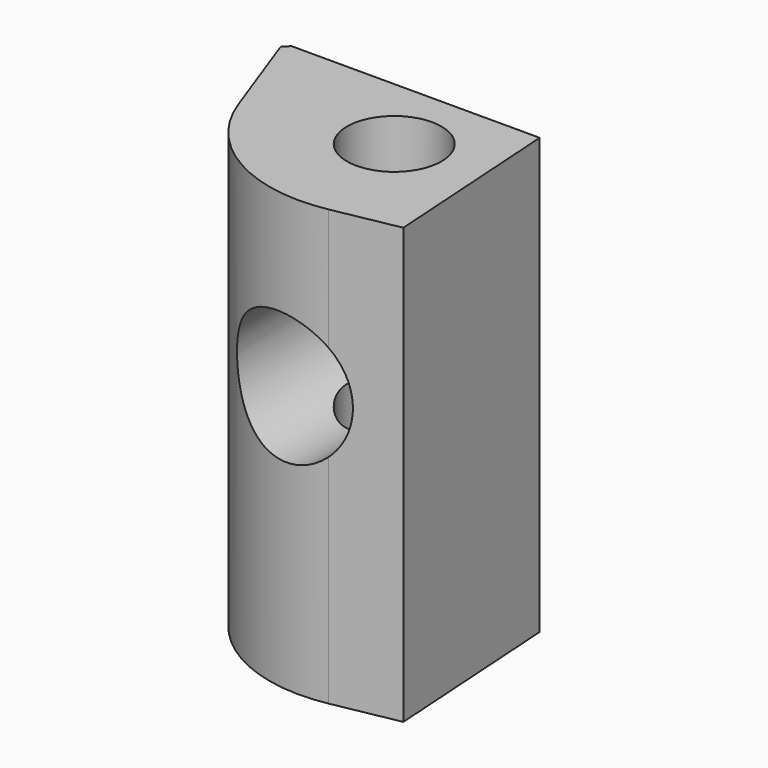
from build123d import *

# Parameters (mm, degrees)
F1_DEPTH    = 74.9545320868
F2_R        = 8.1435947288
F3_DEPTH    = 124.2861971259
F5_R        = 11.2476479719
F6_DEPTH    = 38.057185469
F7_T1_DEPTH = 183.0316575771


# Not quite as in the source:
# - a fillet or chamfer that OpenCascade refuses, or shapes differently, is made with other operations: its cross-section is extruded or revolved along the edge and cut away or added


with BuildPart() as f1:
    # F0 (on Top) → F1 (new body)
    with BuildSketch(Plane.XY):
        Polygon((26.3189487159, 57.2941713035), (-16.4525061846, 57.2941713035), (-17.4609050155, 56.2243200839), (-4.0535703301, 19.2379858345), (28.3696912229, 25.376688689), align=None)
    extrude(amount=F1_DEPTH)

    # F2 (on face) → F3 (cut)
    with BuildSketch(Plane.XY.offset(74.9545320868)):
        with Locations((12.1580604464, 43.6755083501)):
            Circle(F2_R)
    extrude(amount=-F3_DEPTH, mode=Mode.SUBTRACT)

    # F5 (on face) → F6 (cut, through all)
    with BuildSketch(Plane(origin=(0, 57.2941713035, 0), x_dir=(-1, 0, 0), z_dir=(0, 1, 0))):
        with Locations((-9.5685087144, 45.682426542)):
            Circle(F5_R)
    extrude(amount=-F6_DEPTH, mode=Mode.SUBTRACT)

    # F7: fillet of radius 25.4 on 1 edges, made by hand

    # F7_s2 → F7_t1 (cut)
    with BuildSketch(Plane.XY.offset(-54.0385627451)):
        with BuildLine():
            ThreePointArc((17.1845559853, 23.2590047077), (-0.1162411856, 26.147331869), (-11.4199898846, 39.559463761))
            Line((-11.4199898846, 39.559463761), (-4.0535703301, 19.2379858345))
            Line((-4.0535703301, 19.2379858345), (17.1845559853, 23.2590047077))
        make_face()
    extrude(amount=F7_T1_DEPTH, mode=Mode.SUBTRACT)


solid = f1.part
